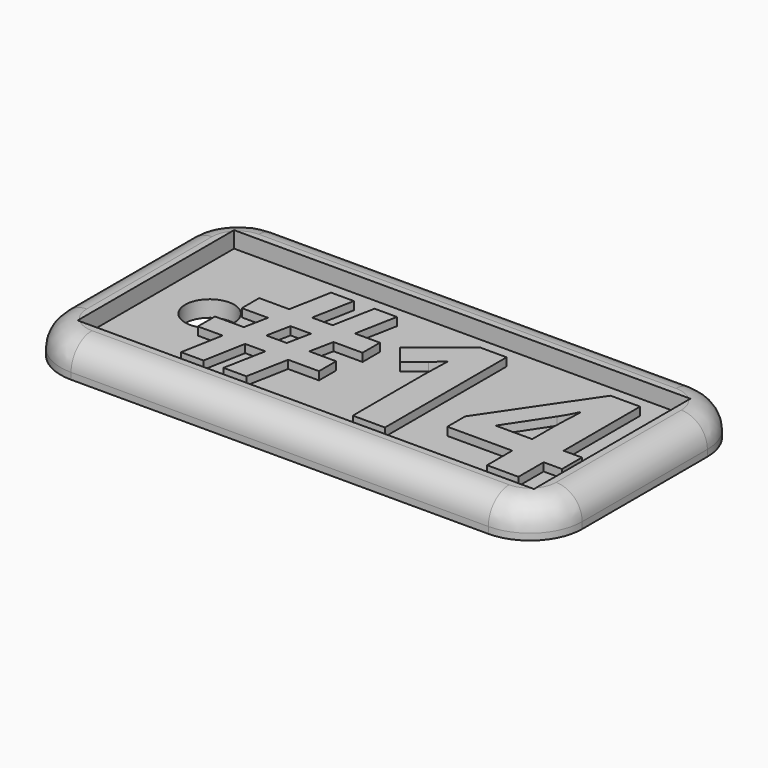
from build123d import *

# Parameters (mm, degrees)
F0_W         = 50.8
F0_H         = 25.4
F0_W_2       = 44.45
F0_H_2       = 19.05
F1_DEPTH     = 3.175
F0_R         = 2.38125
F2_DEPTH     = 1.5875
F3_R         = 5.08
F4_T1_DEPTH  = 40.64
F4_T3_DEPTH  = 15.24
F4_T6_ANGLE  = 90
F4_T8_ANGLE  = 90
F4_T10_ANGLE = 90
F4_T12_ANGLE = 90
F5_TEXT_SIZE = 20.7435133986
F6_DEPTH     = 0.79375


# Not quite as in the source:
# - a fillet or chamfer that OpenCascade refuses, or shapes differently, is made with other operations: its cross-section is extruded or revolved along the edge and cut away or added
# - Text() gives the source's letters only with a copy of the font that has no kerning and outlines rounded to 1/6400 em; it was checked with that copy


with BuildPart() as f1:
    # F0 (on Top) → F1 (new body)
    with BuildSketch(Plane.XY):
        with Locations((25.4, 12.7)):
            Rectangle(F0_W, F0_H)
        with Locations((25.4, 12.7)):
            Rectangle(F0_W_2, F0_H_2, mode=Mode.SUBTRACT)
    extrude(amount=F1_DEPTH)

    # F3
    f3_edges = [f1.edges().sort_by_distance(p)[0] for p in [
        (0, 0, 1.5875),
        (50.8, 0, 1.5875),
        (50.8, 25.4, 1.5875),
        (0, 25.4, 1.5875),
    ]]
    fillet(f3_edges, radius=F3_R)

    # F4: fillet of radius 2.54 on 8 edges, made by hand

    # F4_s2 → F4_t1 (cut)
    with BuildSketch(Plane.YZ.offset(5.08)):
        with BuildLine():
            ThreePointArc((2.54, 3.175), (0.7439487758, 2.4310512242), (0, 0.635))
            Line((0, 0.635), (0, 3.175))
            Line((0, 3.175), (2.54, 3.175))
        make_face()
        with BuildLine():
            ThreePointArc((22.86, 3.175), (24.6560512242, 2.4310512242), (25.4, 0.635))
            Line((25.4, 0.635), (25.4, 3.175))
            Line((25.4, 3.175), (22.86, 3.175))
        make_face()
    extrude(amount=F4_T1_DEPTH, mode=Mode.SUBTRACT)

    # F4_s4 → F4_t3 (cut)
    with BuildSketch(Plane.XZ.offset(-20.32)):
        with BuildLine():
            ThreePointArc((0, 0.635), (0.7439487758, 2.4310512242), (2.54, 3.175))
            Line((2.54, 3.175), (0, 3.175))
            Line((0, 3.175), (0, 0.635))
        make_face()
        with BuildLine():
            ThreePointArc((48.26, 3.175), (50.0560512242, 2.4310512242), (50.8, 0.635))
            Line((50.8, 0.635), (50.8, 3.175))
            Line((50.8, 3.175), (48.26, 3.175))
        make_face()
    extrude(amount=F4_T3_DEPTH, mode=Mode.SUBTRACT)

    # F4_s5 → F4_t6 (revolve, cut)
    with BuildSketch(Plane.XZ.offset(-20.32)):
        with BuildLine():
            ThreePointArc((0, 0.635), (0.7439487758, 2.4310512242), (2.54, 3.175))
            Line((2.54, 3.175), (0, 3.175))
            Line((0, 3.175), (0, 0.635))
        make_face()
    revolve(axis=Axis((5.08, 20.32, 3.175), (0, 0, -1)), revolution_arc=F4_T6_ANGLE, mode=Mode.SUBTRACT)

    # F4_s7 → F4_t8 (revolve, cut)
    with BuildSketch(Plane.XZ.offset(-5.08)):
        with BuildLine():
            ThreePointArc((0, 0.635), (0.7439487758, 2.4310512242), (2.54, 3.175))
            Line((2.54, 3.175), (0, 3.175))
            Line((0, 3.175), (0, 0.635))
        make_face()
    revolve(axis=Axis((5.08, 5.08, 3.175), (0, 0, 1)), revolution_arc=F4_T8_ANGLE, mode=Mode.SUBTRACT)

    # F4_s9 → F4_t10 (revolve, cut)
    with BuildSketch(Plane.XZ.offset(-20.32)):
        with BuildLine():
            ThreePointArc((48.26, 3.175), (50.0560512242, 2.4310512242), (50.8, 0.635))
            Line((50.8, 0.635), (50.8, 3.175))
            Line((50.8, 3.175), (48.26, 3.175))
        make_face()
    revolve(axis=Axis((45.72, 20.32, 3.175), (0, 0, 1)), revolution_arc=F4_T10_ANGLE, mode=Mode.SUBTRACT)

    # F4_s11 → F4_t12 (revolve, cut)
    with BuildSketch(Plane.YZ.offset(45.72)):
        with BuildLine():
            ThreePointArc((2.54, 3.175), (0.7439487758, 2.4310512242), (0, 0.635))
            Line((0, 0.635), (0, 3.175))
            Line((0, 3.175), (2.54, 3.175))
        make_face()
    revolve(axis=Axis((45.72, 5.08, 3.175), (0, 0, 1)), revolution_arc=F4_T12_ANGLE, mode=Mode.SUBTRACT)


with BuildPart() as f2:
    # F0 (on Top) → F2 (new body)
    with BuildSketch(Plane.XY):
        with Locations((25.4, 12.7)):
            Rectangle(F0_W_2, F0_H_2)
        with Locations((8.4216585383, 12.7)):
            Circle(F0_R, mode=Mode.SUBTRACT)
    extrude(amount=F2_DEPTH)

    # F5 (on face) → F6 (join)
    with BuildSketch(Plane.XY.offset(1.5875)):
        with Locations((9.525, 5.1975461882)):
            Text('#14', F5_TEXT_SIZE, font='Open Sans', font_style=FontStyle.BOLD, text_align=(TextAlign.LEFT, TextAlign.BOTTOM))
    extrude(amount=F6_DEPTH)


solid = Compound([f1.part, f2.part])
